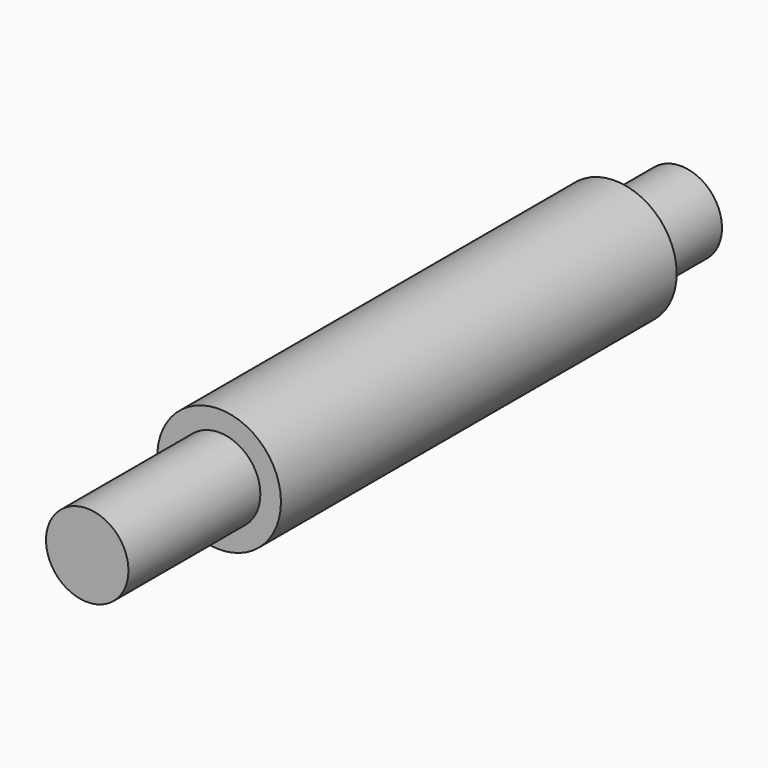
from build123d import *

# Parameters (mm, degrees)
F0_R     = 6.35
F1_DEPTH = 25.4
F2_R     = 9.525
F3_DEPTH = 76.2
F4_R     = 6.35
F5_DEPTH = 12.7


# Not quite as in the source:
# - a feature names something its author has since deleted; it is built from what else it names


with BuildPart() as f1:
    # F0 (on Front) → F1 (new body)
    with BuildSketch(Plane.XZ):
        Circle(F0_R)
    extrude(amount=F1_DEPTH)

    # F2 (on Front) → F3 (join)
    with BuildSketch(Plane.XZ):
        Circle(F2_R)
    extrude(amount=-F3_DEPTH)

    # F4 (on face) → F5 (join)
    with BuildSketch(Plane(origin=(0, 76.2, 0), x_dir=(-1, 0, 0), z_dir=(0, 1, 0))):
        Circle(F4_R)
    extrude(amount=F5_DEPTH)


solid = f1.part
